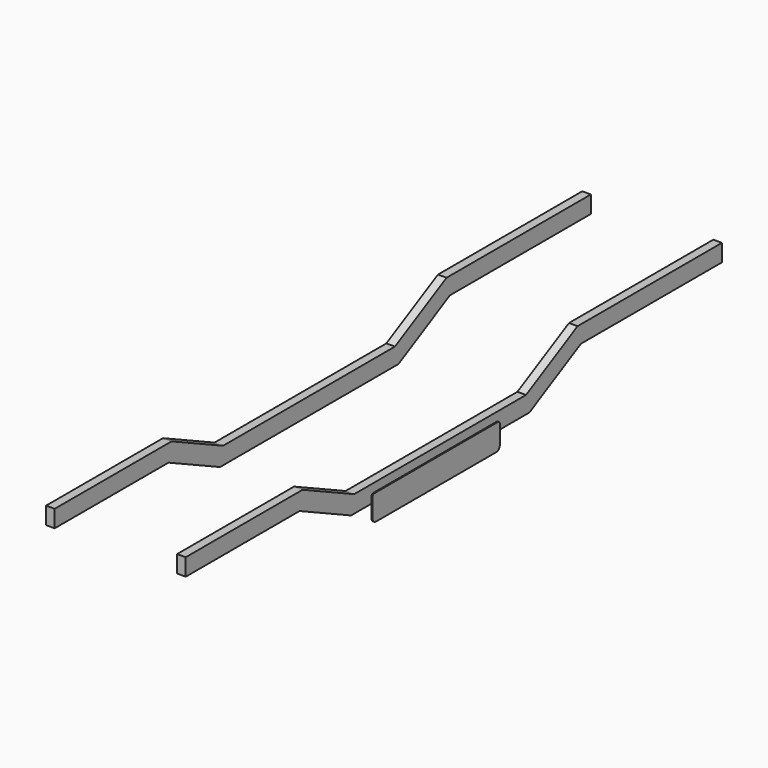
from build123d import *

# Parameters (mm, degrees)
F1_DEPTH = 412.75
F2_W     = 361.95
F2_H     = 4318
F3_DEPTH = 101.601
F4_DEPTH = 203.201
F7_DEPTH = 6.35


# Not quite as in the source:
# - a feature names something its author has since deleted; it is built from what else it names


with BuildPart() as f1:
    # F0 (on Right) → F1 (new body)
    with BuildSketch(Plane.YZ):
        Polygon((-1017.4300536931, 279.4), (-1881.0300536931, 279.4), (-1881.0300536931, 177.8), (-1039.9699463069, 177.8), (-658.9699463069, 0), (658.9699463069, 0), (1039.9699463069, 203.2), (2081.3699463069, 203.2), (2081.3699463069, 304.8), (1014.5699463069, 304.8), (633.5699463069, 101.6), (-636.4300536931, 101.6), align=None)
    extrude(amount=-F1_DEPTH)

    # F2 (on face) → F3 (cut, through all)
    with BuildSketch(Plane.XY.offset(101.6)):
        with Locations((-180.975, 0)):
            Rectangle(F2_W, F2_H)
    extrude(amount=-F3_DEPTH, mode=Mode.SUBTRACT)

    # F2 (on face) → F4 (cut, through all)
    with BuildSketch(Plane.XY.offset(101.6)):
        with Locations((-180.975, 0)):
            Rectangle(F2_W, F2_H)
    extrude(amount=F4_DEPTH, mode=Mode.SUBTRACT)


with BuildPart() as f5_1:
    # F5: instance of F1
    add(f1.part.mirror(Plane.YZ))


with BuildPart() as f7:
    # F6 (on face) → F7 (new body)
    with BuildSketch(Plane.YZ.offset(412.75)):
        with BuildLine():
            Line((419.1, 50.8), (-495.3, 50.8))
            ThreePointArc((-495.3, 50.8), (-504.2802561211, 47.0802561211), (-508, 38.1))
            Line((-508, 38.1), (-508, -76.2))
            ThreePointArc((-508, -76.2), (-500.5605122421, -94.1605122421), (-482.6, -101.6))
            Line((-482.6, -101.6), (406.4, -101.6))
            ThreePointArc((406.4, -101.6), (424.3605122421, -94.1605122421), (431.8, -76.2))
            Line((431.8, -76.2), (431.8, 38.1))
            ThreePointArc((431.8, 38.1), (428.0802561211, 47.0802561211), (419.1, 50.8))
        make_face()
    extrude(amount=F7_DEPTH)


solid = Compound([f1.part, f5_1.part, f7.part])
